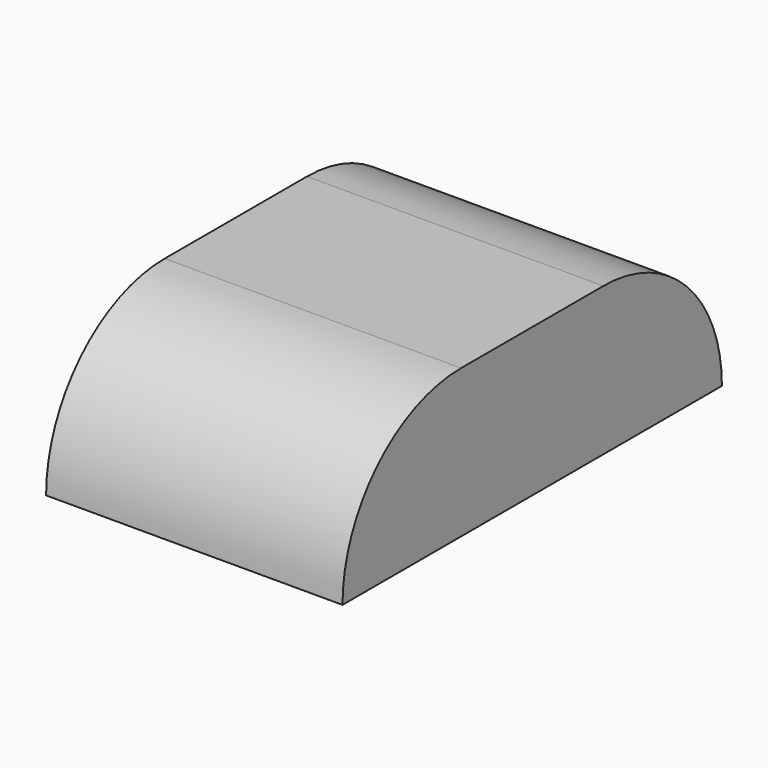
from build123d import *

# Parameters (mm, degrees)
F5_W      = 10
F5_H      = 16
F6_DEPTH  = 5
F0_R      = 1.9
F2_R      = 1.9
F9_R      = 4.99999
F11_DEPTH = 0.2


# Not quite as in the source:
# - a fillet or chamfer is up to 0.001 mm smaller than in the source, because OpenCascade refuses the exact size


with BuildPart() as f6:
    # F5 (on offset) → F6 (new body)
    with BuildSketch(Plane.XY.offset(4.1)):
        with Locations((0, -95.8120375872)):
            Rectangle(F5_W, F5_H)
    extrude(amount=-F6_DEPTH)

    # F0 (on Front) → F7 (revolve, cut)
    with BuildSketch(Plane.XZ):
        with Locations((-92.5, 0)):
            Circle(F0_R)
    revolve(axis=Axis((0, 0, 0), (0, 0, 1)), mode=Mode.SUBTRACT)

    # F2 (on Front) → F8 (revolve, cut)
    with BuildSketch(Plane.XZ):
        with Locations((-100, 0)):
            Circle(F2_R)
    revolve(axis=Axis((0, 0, 0), (0, 0, 1)), mode=Mode.SUBTRACT)

    # F9 (radius 5 in the source; OpenCascade refuses exactly that, so slightly less here)
    f9_edges = [f6.edges().sort_by_distance(p)[0] for p in [
        (0, -103.812038, 4.1),
        (0, -87.812038, 4.1),
    ]]
    fillet(f9_edges, radius=F9_R)

    # F10 (on face) → F11 (join)
    with BuildSketch(Plane.YZ.offset(5)):
        with BuildLine():
            Line((-92.8120375872, 4.1), (-98.8120375872, 4.1))
            ThreePointArc((-98.8120375872, 4.1), (-102.3475714931, 2.6355339059), (-103.8120375872, -0.9))
            Line((-103.8120375872, -0.9), (-87.8120375872, -0.9))
            ThreePointArc((-87.8120375872, -0.9), (-89.2765036812, 2.6355339059), (-92.8120375872, 4.1))
        make_face()
    extrude(amount=-F11_DEPTH)


solid = f6.part
